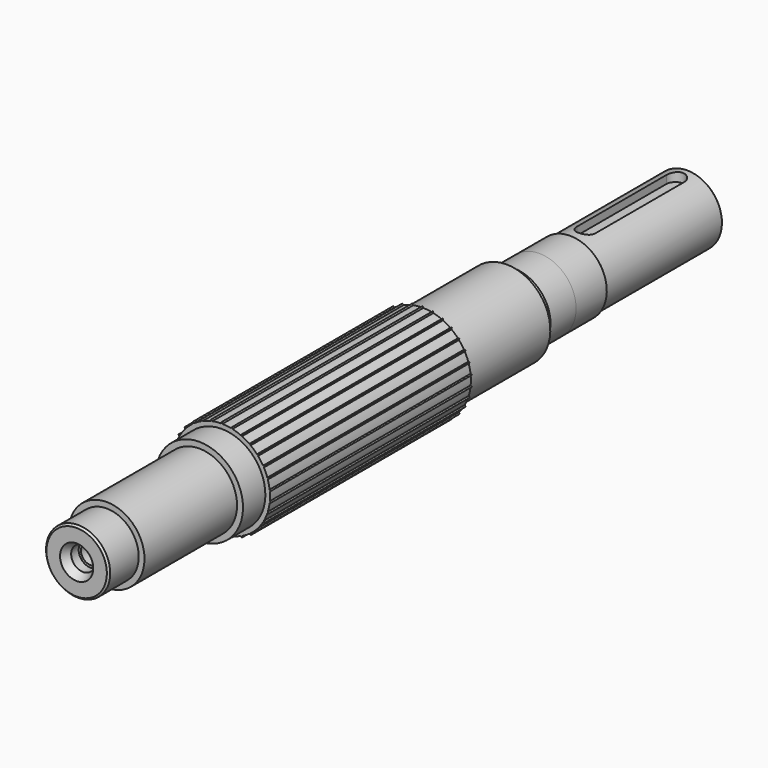
from build123d import *

# Parameters (mm, degrees)
F3_DEPTH        = 235.8934182005
F3_COPIES_COUNT = 30
F6_DEPTH        = 5
F7_SIZE         = 1.016
F10_D           = 10.5
F10_DEPTH       = 31.9574
F10_TIP         = 3.1545182499
F11_SIZE        = 0.762
F14_D           = 10.5
F14_DEPTH       = 31.9532
F14_TIP         = 3.1545182499


# Not quite as in the source:
# - a pattern or mirror of a feature is missing from the dataset's text; its kind, count and spacing are read off the source's solid


with BuildPart() as f1:
    # F0 (on Right) → F1 (revolve)
    with BuildSketch(Plane.YZ):
        with BuildLine():
            Line((59.3317817995, 23.876), (2.032, 23.876))
            Line((2.032, 23.876), (2.032, 27.1526))
            Line((2.032, 27.1526), (0, 27.1526))
            Line((0, 27.1526), (-135, 27.1526))
            Line((-135, 27.1526), (-135, 23.876))
            Line((-135, 23.876), (-150.24, 23.876))
            Line((-150.24, 23.876), (-150.24, 20.6375))
            Line((-150.24, 20.6375), (-213.3880182005, 20.6375))
            Line((-213.3880182005, 20.6375), (-213.3880182005, 17.5006))
            Line((-213.3880182005, 17.5006), (-233.8604182005, 17.5006))
            Line((-233.8604182005, 17.5006), (-233.8604182005, 9.0551))
            Line((-233.8604182005, 9.0551), (-229.4662182005, 6.5024))
            Line((-229.4662182005, 6.5024), (-224.3608182005, 6.5024))
            Line((-224.3608182005, 6.5024), (-224.3608182005, 0))
            Line((-224.3608182005, 0), (174.0127817995, 0))
            Line((174.0127817995, 0), (174.0127817995, 6.5024))
            Line((174.0127817995, 6.5024), (179.1181817995, 6.5024))
            Line((179.1181817995, 6.5024), (183.5123817995, 9.0551))
            Line((183.5123817995, 9.0551), (183.5123817995, 18.9992))
            Line((183.5123817995, 18.9992), (103.5023817995, 18.9992))
            Line((103.5023817995, 18.9992), (103.5023817995, 19.97075))
            Line((103.5023817995, 19.97075), (81.7853817995, 19.97075))
            Line((81.7853817995, 19.97075), (81.7853817995, 20.00758))
            Line((81.7853817995, 20.00758), (64.3216122695, 20.00758))
            Line((64.3216122695, 20.00758), (62.6845817995, 19.0624400175))
            ThreePointArc((62.6845817995, 19.0624400175), (60.4493817995, 19.0624400175), (59.3317817995, 20.99818))
            Line((59.3317817995, 20.99818), (59.3317817995, 23.876))
        make_face()
    revolve(axis=Axis((0, -25.1740182005, 0), (0, 1, 0)))

    # F2 (on face) → F3 (cut, through all)
    with BuildSketch(Plane(origin=(0, 2.032, 0), x_dir=(-1, 0, 0), z_dir=(0, 1, 0))):
        with BuildLine():
            Line((-0.442078818, 26.3868970263), (0, 27.1526))
            ThreePointArc((0, 27.1526), (-2.8382195517, 27.0038552162), (-5.6453429761, 26.5592505437))
            Line((-5.6453429761, 26.5592505437), (-5.0537260411, 25.9021933716))
            ThreePointArc((-5.0537260411, 25.9021933716), (-2.7585688627, 26.2460295319), (-0.442078818, 26.3868970263))
        make_face()
    f3 = extrude(amount=-F3_DEPTH, mode=Mode.SUBTRACT)

    # F3_copies: F3 ×30 about axis
    f3_copies_axis = Axis((0, 0, 0), (0, 1, 0))
    for i in range(1, F3_COPIES_COUNT):
        add(f3.rotate(f3_copies_axis, i * 360 / F3_COPIES_COUNT), mode=Mode.SUBTRACT)

    # F5 (on offset) → F6 (cut)
    with BuildSketch(Plane.XY.offset(18.9992)):
        with BuildLine():
            Line((-4.99999, 174.5207817995), (-4.99999, 113.5607817995))
            ThreePointArc((-4.99999, 113.5607817995), (0, 108.5607917995), (4.99999, 113.5607817995))
            Line((4.99999, 113.5607817995), (4.99999, 174.5207817995))
            ThreePointArc((4.99999, 174.5207817995), (0, 179.5207717995), (-4.99999, 174.5207817995))
        make_face()
    extrude(amount=-F6_DEPTH, mode=Mode.SUBTRACT)

    # F7
    f7_edges = [f1.edges().sort_by_distance(p)[0] for p in [
        (0, 183.512382, -18.9992),
        (0, -233.860418, -17.5006),
    ]]
    chamfer(f7_edges, length=F7_SIZE)

    # F10
    with Locations(Plane(origin=(0, 174.0127817995, 0), x_dir=(-1, 0, 0), z_dir=(0, 1, 0))):
        with Locations((0, 0)):
            Hole(F10_D / 2, depth=F10_DEPTH)
            with Locations((0, 0, -(F10_DEPTH + F10_TIP / 2))):  # 118° drill point
                Cone(0, F10_D / 2, F10_TIP, mode=Mode.SUBTRACT)

    # F11
    f11_edges = [f1.edges().sort_by_distance(p)[0] for p in [
        (0, 103.502382, -19.97075),
    ]]
    chamfer(f11_edges, length=F11_SIZE)

    # F14
    with Locations(Plane.XZ.offset(224.3608182005)):
        with Locations((0, 0)):
            Hole(F14_D / 2, depth=F14_DEPTH)
            with Locations((0, 0, -(F14_DEPTH + F14_TIP / 2))):  # 118° drill point
                Cone(0, F14_D / 2, F14_TIP, mode=Mode.SUBTRACT)


solid = f1.part
